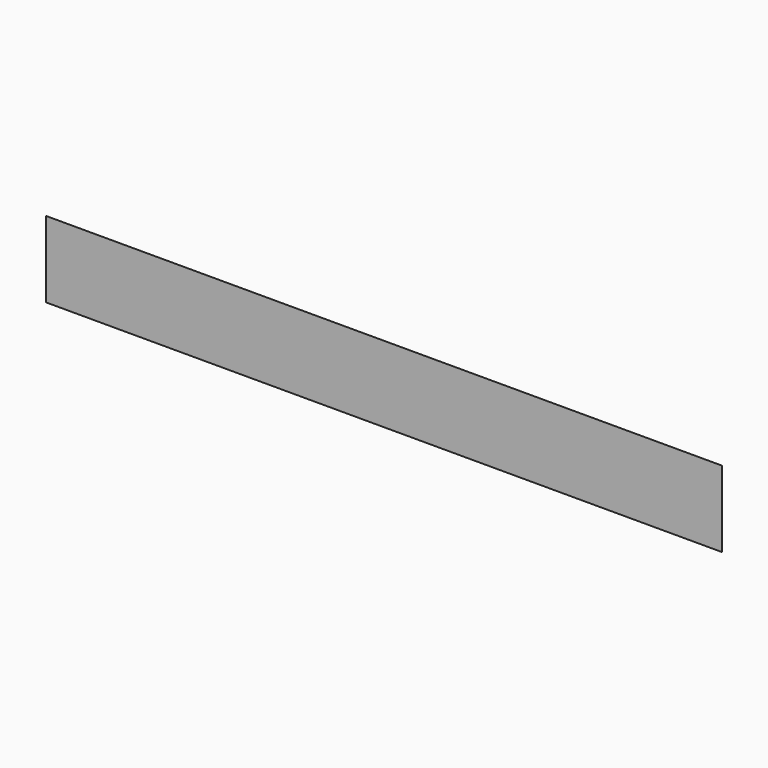
from build123d import *

# Parameters (mm, degrees)
F0_W     = 2311.4
F0_H     = 260.35
F1_DEPTH = 19.05
F2_SIZE  = 19.04999


# Not quite as in the source:
# - a fillet or chamfer is up to 0.001 mm smaller than in the source, because OpenCascade refuses the exact size


with BuildPart() as f1:
    # F0 (on Front) → F1 (new body)
    with BuildSketch(Plane.XZ):
        Rectangle(F0_W, F0_H)
    extrude(amount=F1_DEPTH)

    # F2 (size 19.05 in the source; OpenCascade refuses exactly that, so slightly less here)
    f2_edges = [f1.edges().sort_by_distance(p)[0] for p in [
        (1155.7, 0, 0),
        (0, 0, 130.175),
        (-1155.7, 0, 0),
        (0, 0, -130.175),
    ]]
    chamfer(f2_edges, length=F2_SIZE)


solid = f1.part
